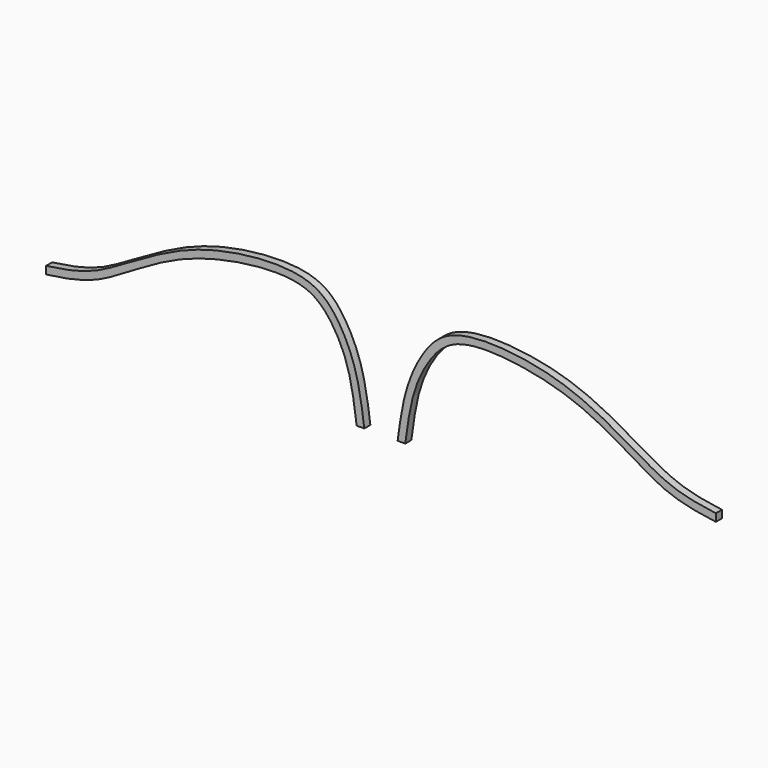
from build123d import *

# Parameters (mm, degrees)
F1_DEPTH = 1.5875


# Not quite as in the source:
# - a length typed as a fraction of an inch, garbled in the dataset ("3 / 203.2 mm" for 3/8 in), is restored


with BuildPart() as f1:
    # F0 (on Front) → F1 (new body)
    with BuildSketch(Plane.XZ):
        with BuildLine():
            add(Edge.make_bspline(
                [(-69.8618200234, -4.0307355407), (-62.7915279521, -3.1209299924), (-57.2238344828, -0.8035358429), (-44.0257855414, 7.5637777447), (-30.9070015059, 11.7718739084), (-15.0047259193, 12.4340705831), (-8.7446333351, 6.2657200791), (-4.6801867065, -2.5297780334), (-3.8012916914, -9.9607688029), (-3.4819712574, -12.3153160934)],
                knots=[0, 0, 0, 0, 0.1547177739, 0.3097210327, 0.4672770518, 0.6266889873, 0.7429785033, 0.8723441321, 1, 1, 1, 1], degree=3))
            Line((-69.8618200234, -4.0307355407), (-69.8618200234, -5.6182355407))
            add(Edge.make_bspline(
                [(-5.0694712574, -12.3153160934), (-5.3867439208, -10.0413757398), (-6.2604337301, -2.5037762179), (-10.0520808031, 5.206448905), (-15.7989784307, 10.9471177854), (-30.5114508321, 10.1394782106), (-44.1256162236, 6.0468191153), (-56.8318396104, -2.4198026522), (-62.6670705525, -4.7084299924), (-69.8618200234, -5.6182355407)],
                knots=[0, 0, 0, 0, 0.1297378292, 0.2541417516, 0.3670013899, 0.5229680625, 0.6851275071, 0.8410548588, 1, 1, 1, 1], degree=3))
            Line((-5.0694712574, -12.3153160934), (-3.4819712574, -12.3153160934))
        make_face()
    extrude(amount=F1_DEPTH)


with BuildPart() as f1b:
    # F0 (on Front) → F1, piece 2 (new body)
    with BuildSketch(Plane.XZ):
        with BuildLine():
            Line((69.8618200234, -5.6182355407), (69.8618200234, -4.0307355407))
            add(Edge.make_bspline(
                [(69.8618200234, -4.0307355407), (62.7915279521, -3.1209299924), (57.2238344828, -0.8035358429), (44.0257855414, 7.5637777447), (30.9070015059, 11.7718739084), (15.0047259193, 12.4340705831), (8.7446333351, 6.2657200791), (4.6801867065, -2.5297780334), (3.8012916914, -9.9607688029), (3.4819712574, -12.3153160934)],
                knots=[0, 0, 0, 0, 0.1547177739, 0.3097210327, 0.4672770518, 0.6266889873, 0.7429785033, 0.8723441321, 1, 1, 1, 1], degree=3))
            Line((3.4819712574, -12.3153160934), (5.0694712574, -12.3153160934))
            add(Edge.make_bspline(
                [(5.0694712574, -12.3153160934), (5.3867439208, -10.0413757398), (6.2604337301, -2.5037762179), (10.0520808031, 5.206448905), (15.7989784307, 10.9471177854), (30.5114508321, 10.1394782106), (44.1256162236, 6.0468191153), (56.8318396104, -2.4198026522), (62.6670705525, -4.7084299924), (69.8618200234, -5.6182355407)],
                knots=[0, 0, 0, 0, 0.1297378292, 0.2541417516, 0.3670013899, 0.5229680625, 0.6851275071, 0.8410548588, 1, 1, 1, 1], degree=3))
        make_face()
    extrude(amount=F1_DEPTH)


solid = Compound([f1.part, f1b.part])
